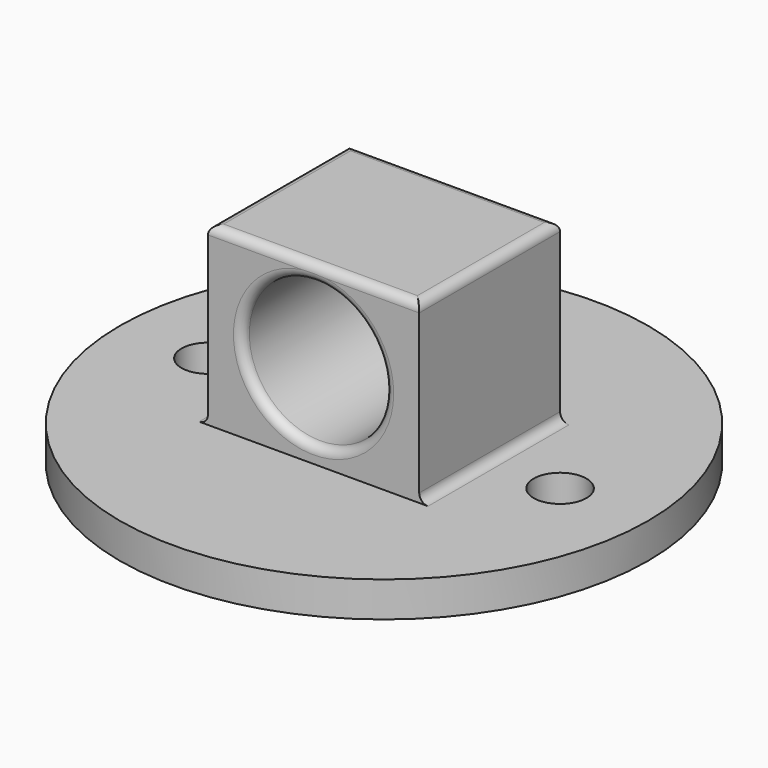
from build123d import *

# Parameters (mm, degrees)
F0_R        = 15
F1_DEPTH    = 2
F2_W        = 12
F2_H        = 10
F3_DEPTH    = 10
F4_R        = 4.05
F5_DEPTH    = 20.001
F6_R        = 1.5
F7_DEPTH    = 2.001
F8_T1_DEPTH = 10
F8_T3_DEPTH = 14.5
F8_T5_DEPTH = 12.5


# Not quite as in the source:
# - a fillet or chamfer that OpenCascade refuses, or shapes differently, is made with other operations: its cross-section is extruded or revolved along the edge and cut away or added


with BuildPart() as f1:
    # F0 (on Top) → F1 (new body)
    with BuildSketch(Plane.XY):
        Circle(F0_R)
    extrude(amount=F1_DEPTH)

    # F2 (on face) → F3 (join)
    with BuildSketch(Plane.XY.offset(2)):
        Rectangle(F2_W, F2_H)
    extrude(amount=F3_DEPTH)

    # F4 (on face) → F5 (cut, through all)
    with BuildSketch(Plane.XZ.offset(5)):
        with Locations((0, 7)):
            Circle(F4_R)
    extrude(amount=-F5_DEPTH, mode=Mode.SUBTRACT)

    # F6 (on face) → F7 (cut, through all)
    with BuildSketch(Plane.XY.offset(2)):
        with Locations((10, 0)):
            Circle(F6_R)
        with Locations((-10, 0)):
            Circle(F6_R)
    extrude(amount=-F7_DEPTH, mode=Mode.SUBTRACT)

    # F8: fillet of radius 0.5 on 8 edges, made by hand

    # F8_s2 → F8_t1 (join)
    with BuildSketch(Plane.XZ.offset(-5)):
        with BuildLine():
            ThreePointArc((-6.5, 2), (-6.1464466094, 2.1464466094), (-6, 2.5))
            Line((-6, 2.5), (-6, 2))
            Line((-6, 2), (-6.5, 2))
        make_face()
        with BuildLine():
            ThreePointArc((6.5, 2), (6.1464466094, 2.1464466094), (6, 2.5))
            Line((6, 2.5), (6, 2))
            Line((6, 2), (6.5, 2))
        make_face()
    extrude(amount=F8_T1_DEPTH)

    # F8_s4 → F8_t3 (cut)
    with BuildSketch(Plane.YZ.offset(-7.25)):
        with BuildLine():
            ThreePointArc((-4.5, 12), (-4.8535533906, 11.8535533906), (-5, 11.5))
            Line((-5, 11.5), (-5, 12))
            Line((-5, 12), (-4.5, 12))
        make_face()
        with BuildLine():
            ThreePointArc((4.5, 12), (4.8535533906, 11.8535533906), (5, 11.5))
            Line((5, 11.5), (5, 12))
            Line((5, 12), (4.5, 12))
        make_face()
    extrude(amount=F8_T3_DEPTH, mode=Mode.SUBTRACT)

    # F8_s6 → F8_t5 (cut)
    with BuildSketch(Plane.XZ.offset(-6.25)):
        with BuildLine():
            ThreePointArc((5.5, 12), (5.8535533906, 11.8535533906), (6, 11.5))
            Line((6, 11.5), (6, 12))
            Line((6, 12), (5.5, 12))
        make_face()
        with BuildLine():
            ThreePointArc((-6, 11.5), (-5.8535533906, 11.8535533906), (-5.5, 12))
            Line((-5.5, 12), (-6, 12))
            Line((-6, 12), (-6, 11.5))
        make_face()
    extrude(amount=F8_T5_DEPTH, mode=Mode.SUBTRACT)

    # F8_s7 → F8_t8 (revolve, cut)
    with BuildSketch(Plane.XY.offset(7)):
        with BuildLine():
            ThreePointArc((4.05, 4.5), (4.1964466094, 4.8535533906), (4.55, 5))
            Line((4.55, 5), (4.05, 5))
            Line((4.05, 5), (4.05, 4.5))
        make_face()
    revolve(axis=Axis((0, 5, 7), (0, -1, 0)), mode=Mode.SUBTRACT)

    # F8_s9 → F8_t10 (revolve, cut)
    with BuildSketch(Plane.XY.offset(7)):
        with BuildLine():
            ThreePointArc((4.55, -5), (4.1964466094, -4.8535533906), (4.05, -4.5))
            Line((4.05, -4.5), (4.05, -5))
            Line((4.05, -5), (4.55, -5))
        make_face()
    revolve(axis=Axis((0, -5, 7), (0, -1, 0)), mode=Mode.SUBTRACT)


solid = f1.part
